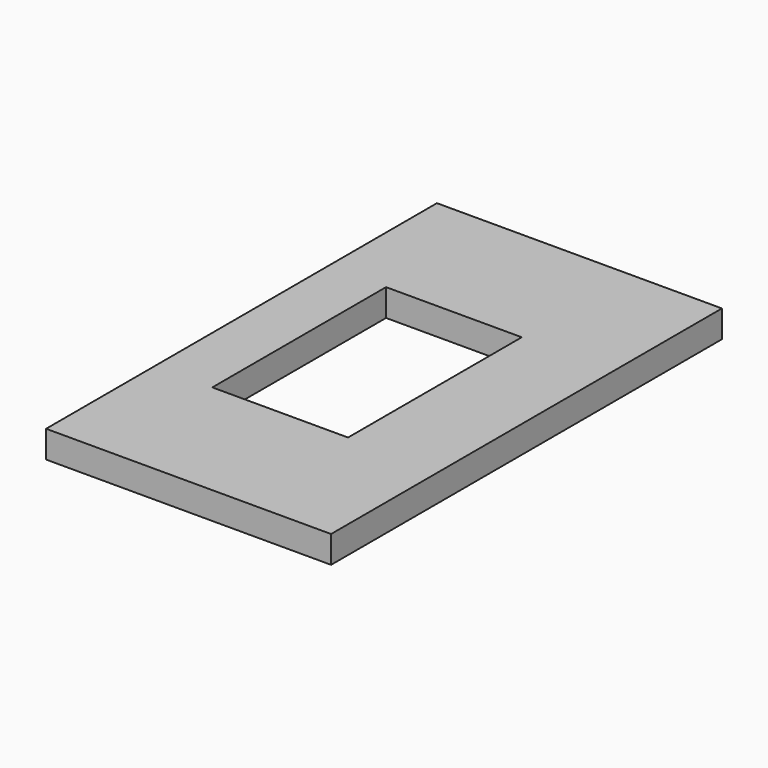
from build123d import *

# Parameters (mm, degrees)
F0_W     = 42
F0_H     = 72
F1_DEPTH = 4


# Not quite as in the source:
# - ends of sketch curves that miss each other by under 0.0002 mm in the source are joined


with BuildPart() as f1:
    # F0 (on Top) → F1 (new body)
    with BuildSketch(Plane.XY):
        Rectangle(F0_W, F0_H)
        Polygon((-12.5, -16), (-12.5, 16), (7.5, 16), (7.4999813996, -15.999997206), align=None, mode=Mode.SUBTRACT)
    extrude(amount=F1_DEPTH)


solid = f1.part
